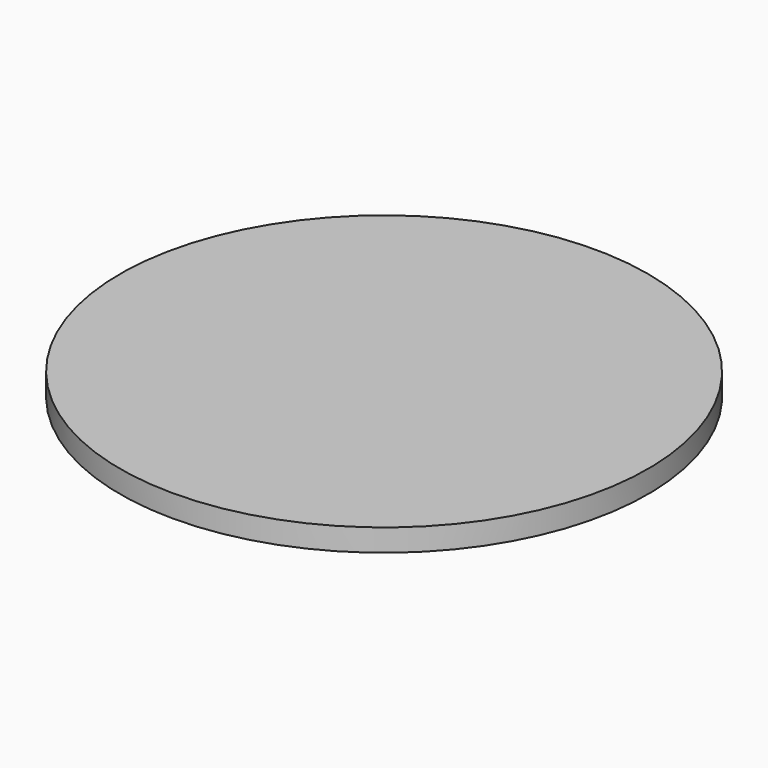
from build123d import *

# Parameters (mm, degrees)
F4_W = 94.9315726757
F4_H = 8.022087859
F7_T = -5.08


# Not quite as in the source:
# - the program builds the solid bodies; features that only make, move or delete a surface that nothing else refers to are left out


with BuildPart() as f6:
    # F4 (on Right) → F6 (revolve)
    with BuildSketch(Plane.YZ):
        with Locations((-47.4657863379, -0.8492631605)):
            Rectangle(F4_W, F4_H)
    revolve(axis=Axis((0, 0, -18.7146086246), (0, 0, -1)))

    # F7
    f7_openings = [f6.faces().sort_by_distance(p)[0] for p in [
        (0, 0, -4.860307),
    ]]
    offset(amount=F7_T, openings=f7_openings)


solid = f6.part
